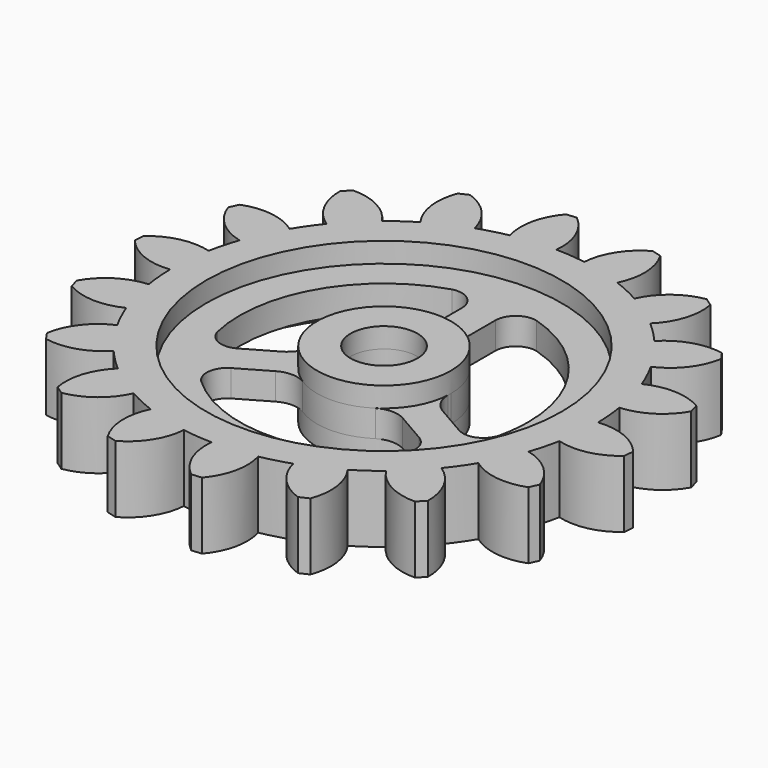
from build123d import *
from build123d import SkipClean  # not in build123d's __all__

# Parameters (mm, degrees)
F2_R      = 2.5
F4_DEPTH  = 5
F5_COUNT  = 18
F5_ANGLE  = 340
F7_DEPTH  = 5.001
F6_R      = 13.27
F6_W      = 2.5
F6_H      = 2.618576711
F8_DEPTH  = 1.5
F9_DEPTH  = 5.001
F10_START = 3.5
F10_DEPTH = 1.5
F11_R     = 5
F11_R_2   = 2.5
F12_DEPTH = 5


# Not quite as in the source:
# - a feature names something its author has since deleted; it is built from what else it names


with BuildPart() as f4:
    # F2 (on Top) → F4 (new body)
    with BuildSketch(Plane.XY):
        with BuildLine():
            ThreePointArc((-2.990858108, 15.4837872556), (-1.3744460631, 15.7099903889), (0.2566888126, 15.7679107955))
            ThreePointArc((0.2566888126, 15.7679107955), (-0.0491419998, 17.9196352526), (-1.341787956, 19.666780655))
            Line((-1.341787956, 19.666780655), (-2.0936974393, 19.6009970992))
            ThreePointArc((-2.0936974393, 19.6009970992), (-3.0633165837, 17.6559291466), (-2.990858108, 15.4837872556))
        make_face()
        with BuildLine():
            ThreePointArc((-2.990858108, 15.4837872556), (-10.0381040948, -12.1626216821), (15.77, 0))
            ThreePointArc((15.77, 0), (11.2414608164, 11.0599484046), (0.2566888126, 15.7679107955))
            ThreePointArc((0.2566888126, 15.7679107955), (-1.3744460631, 15.7099903889), (-2.990858108, 15.4837872556))
        make_face()
        Circle(F2_R, mode=Mode.SUBTRACT)
    extrude(amount=F4_DEPTH)

    # F5: F4 ×18 about axis
    f5_axis = Axis((0, 0, 30.7848658413), (0, 0, 1))


with BuildPart() as f4_1:
    add(f4.part, clean=False)
    for i in range(1, F5_COUNT):
        add(f4.part.rotate(f5_axis, i * F5_ANGLE / (F5_COUNT - 1)), clean=False)

    # F6 (on Top) → F7 (cut, through all)
    with BuildSketch(Plane.XY):
        with BuildLine():
            ThreePointArc((2.2618683613, 4.4591424642), (4.2608298374, 2.6163579833), (5, 0))
            ThreePointArc((5, 0), (4.9981658722, -0.1354175543), (4.9926648344, -0.2707357593))
            ThreePointArc((4.9926648344, -0.2707357593), (5.2571580162, -1.2784847908), (5.9926180702, -2.0164639659))
            Line((5.9926180702, -2.0164639659), (8.2603720268, -3.325752316))
            ThreePointArc((8.2603720268, -3.325752316), (9.5998090611, -3.4180506459), (10.4951545309, -2.4175672426))
            ThreePointArc((10.4951545309, -2.4175672426), (10.7010680378, -1.2165701176), (10.77, 0))
            ThreePointArc((10.77, 0), (8.6591117019, 6.4041146566), (3.1539025934, 10.2978540692))
            ThreePointArc((3.1539025934, 10.2978540692), (1.8397858158, 10.0227038458), (1.25, 8.8165681809))
            Line((1.25, 8.8165681809), (1.25, 6.1979914699))
            ThreePointArc((1.25, 6.1979914699), (1.5213786885, 5.1920747928), (2.2618683613, 4.4591424642))
        make_face()
        with BuildLine():
            ThreePointArc((-4.9926648325, -0.2707357951), (-4.3301270249, 2.4999999896), (-2.2618683613, 4.4591424642))
            ThreePointArc((-2.2618683613, 4.4591424642), (-1.5213786885, 5.1920747928), (-1.25, 6.1979914699))
            Line((-1.25, 6.1979914699), (-1.25, 8.8165681809))
            ThreePointArc((-1.25, 8.8165681809), (-1.8397858158, 10.0227038458), (-3.1539025934, 10.2978540692))
            ThreePointArc((-3.1539025934, 10.2978540692), (-9.3270936116, 5.3849999777), (-10.4951545136, -2.4175673179))
            ThreePointArc((-10.4951545136, -2.4175673179), (-9.5998090366, -3.4180507148), (-8.260372003, -3.3257523753))
            Line((-8.260372003, -3.3257523753), (-5.9926180557, -2.0164640089))
            ThreePointArc((-5.9926180557, -2.0164640089), (-5.257158007, -1.2784848286), (-4.9926648325, -0.2707357951))
        make_face()
    extrude(amount=F7_DEPTH, mode=Mode.SUBTRACT)

    # F6 (on Top) → F8 (cut)
    with BuildSketch(Plane.XY):
        Circle(F6_R)
        with BuildLine():
            ThreePointArc((-3.1539025934, 10.2978540692), (0, 10.77), (3.1539025934, 10.2978540692))
            ThreePointArc((3.1539025934, 10.2978540692), (8.6591117019, 6.4041146566), (10.77, 0))
            ThreePointArc((10.77, 0), (10.7010680378, -1.2165701176), (10.4951545309, -2.4175672426))
            ThreePointArc((10.4951545309, -2.4175672426), (9.3270936116, -5.3849999777), (7.3412519506, -7.880286784))
            ThreePointArc((7.3412519506, -7.880286784), (3.87e-08, -10.77), (-7.341251894, -7.8802868367))
            ThreePointArc((-7.341251894, -7.8802868367), (-9.327093573, -5.3850000446), (-10.4951545136, -2.4175673179))
            ThreePointArc((-10.4951545136, -2.4175673179), (-9.3270936116, 5.3849999777), (-3.1539025934, 10.2978540692))
        make_face(mode=Mode.SUBTRACT)
        with BuildLine():
            ThreePointArc((4.9926648344, -0.2707357593), (4.9981658722, -0.1354175543), (5, 0))
            ThreePointArc((5, 0), (4.2608298374, 2.6163579833), (2.2618683613, 4.4591424642))
            ThreePointArc((2.2618683613, 4.4591424642), (0, 5), (-2.2618683613, 4.4591424642))
            ThreePointArc((-2.2618683613, 4.4591424642), (-4.3301270249, 2.4999999896), (-4.9926648325, -0.2707357951))
            ThreePointArc((-4.9926648325, -0.2707357951), (-4.330127007, -2.5000000207), (-2.7307964524, -4.1884067061))
            ThreePointArc((-2.7307964524, -4.1884067061), (1.79e-08, -5), (2.7307964825, -4.1884066865))
            ThreePointArc((2.7307964825, -4.1884066865), (4.3301270249, -2.4999999896), (4.9926648344, -0.2707357593))
        make_face()
        with BuildLine():
            ThreePointArc((-2.2618683613, 4.4591424642), (0, 5), (2.2618683613, 4.4591424642))
            ThreePointArc((2.2618683613, 4.4591424642), (1.5213786885, 5.1920747928), (1.25, 6.1979914699))
            Line((1.25, 6.1979914699), (-1.25, 6.1979914699))
            ThreePointArc((-1.25, 6.1979914699), (-1.5213786885, 5.1920747928), (-2.2618683613, 4.4591424642))
        make_face()
        with Locations((0, 7.5072798254)):
            Rectangle(F6_W, F6_H)
        with BuildLine():
            Line((-1.25, 8.8165681809), (1.25, 8.8165681809))
            ThreePointArc((1.25, 8.8165681809), (1.8397858158, 10.0227038458), (3.1539025934, 10.2978540692))
            ThreePointArc((3.1539025934, 10.2978540692), (0, 10.77), (-3.1539025934, 10.2978540692))
            ThreePointArc((-3.1539025934, 10.2978540692), (-1.8397858158, 10.0227038458), (-1.25, 8.8165681809))
        make_face()
        with BuildLine():
            ThreePointArc((-2.7307964524, -4.1884067061), (-4.330127007, -2.5000000207), (-4.9926648325, -0.2707357951))
            ThreePointArc((-4.9926648325, -0.2707357951), (-5.257158007, -1.2784848286), (-5.9926180557, -2.0164640089))
            Line((-5.9926180557, -2.0164640089), (-4.7426180454, -4.1815275124))
            ThreePointArc((-4.7426180454, -4.1815275124), (-3.7357793059, -3.9135900073), (-2.7307964524, -4.1884067061))
        make_face()
        Polygon((-4.7426180454, -4.1815275124), (-5.9926180557, -2.0164640089), (-8.260372003, -3.3257523753), (-7.0103719926, -5.4908158787), align=None)
        with BuildLine():
            Line((-7.0103719926, -5.4908158787), (-8.260372003, -3.3257523753))
            ThreePointArc((-8.260372003, -3.3257523753), (-9.5998090366, -3.4180507148), (-10.4951545136, -2.4175673179))
            ThreePointArc((-10.4951545136, -2.4175673179), (-9.327093573, -5.3850000446), (-7.341251894, -7.8802868367))
            ThreePointArc((-7.341251894, -7.8802868367), (-7.7600232055, -6.6046532141), (-7.0103719926, -5.4908158787))
        make_face()
        with BuildLine():
            ThreePointArc((10.4951545309, -2.4175672426), (9.5998090611, -3.4180506459), (8.2603720268, -3.325752316))
            Line((8.2603720268, -3.325752316), (7.010372032, -5.4908158284))
            ThreePointArc((7.010372032, -5.4908158284), (7.7600232529, -6.6046531583), (7.3412519506, -7.880286784))
            ThreePointArc((7.3412519506, -7.880286784), (9.3270936116, -5.3849999777), (10.4951545309, -2.4175672426))
        make_face()
        Polygon((8.2603720268, -3.325752316), (5.9926180702, -2.0164639659), (4.7426180754, -4.1815274783), (7.010372032, -5.4908158284), align=None)
        with BuildLine():
            ThreePointArc((5.9926180702, -2.0164639659), (5.2571580162, -1.2784847908), (4.9926648344, -0.2707357593))
            ThreePointArc((4.9926648344, -0.2707357593), (4.3301270249, -2.4999999896), (2.7307964825, -4.1884066865))
            ThreePointArc((2.7307964825, -4.1884066865), (3.735779334, -3.9135899804), (4.7426180754, -4.1815274783))
            Line((4.7426180754, -4.1815274783), (5.9926180702, -2.0164639659))
        make_face()
    extrude(amount=F8_DEPTH, mode=Mode.SUBTRACT)

    # F9 (cut, through all): a face of the model
    f9_faces = [f4_1.faces().sort_by_distance(p)[0] for p in [
        (2.61e-08, -7.2727720269, 0),
    ]]
    extrude(f9_faces, amount=-F9_DEPTH, mode=Mode.SUBTRACT)

    # F6 (on Top) → F10 (cut)
    with BuildSketch(Plane.XY.offset(F10_START)):
        Circle(F6_R)
        with BuildLine():
            ThreePointArc((-3.1539025934, 10.2978540692), (0, 10.77), (3.1539025934, 10.2978540692))
            ThreePointArc((3.1539025934, 10.2978540692), (8.6591117019, 6.4041146566), (10.77, 0))
            ThreePointArc((10.77, 0), (10.7010680378, -1.2165701176), (10.4951545309, -2.4175672426))
            ThreePointArc((10.4951545309, -2.4175672426), (9.3270936116, -5.3849999777), (7.3412519506, -7.880286784))
            ThreePointArc((7.3412519506, -7.880286784), (3.87e-08, -10.77), (-7.341251894, -7.8802868367))
            ThreePointArc((-7.341251894, -7.8802868367), (-9.327093573, -5.3850000446), (-10.4951545136, -2.4175673179))
            ThreePointArc((-10.4951545136, -2.4175673179), (-9.3270936116, 5.3849999777), (-3.1539025934, 10.2978540692))
        make_face(mode=Mode.SUBTRACT)
        with BuildLine():
            ThreePointArc((4.9926648344, -0.2707357593), (4.9981658722, -0.1354175543), (5, 0))
            ThreePointArc((5, 0), (4.2608298374, 2.6163579833), (2.2618683613, 4.4591424642))
            ThreePointArc((2.2618683613, 4.4591424642), (0, 5), (-2.2618683613, 4.4591424642))
            ThreePointArc((-2.2618683613, 4.4591424642), (-4.3301270249, 2.4999999896), (-4.9926648325, -0.2707357951))
            ThreePointArc((-4.9926648325, -0.2707357951), (-4.330127007, -2.5000000207), (-2.7307964524, -4.1884067061))
            ThreePointArc((-2.7307964524, -4.1884067061), (1.79e-08, -5), (2.7307964825, -4.1884066865))
            ThreePointArc((2.7307964825, -4.1884066865), (4.3301270249, -2.4999999896), (4.9926648344, -0.2707357593))
        make_face()
        with BuildLine():
            ThreePointArc((10.4951545309, -2.4175672426), (9.5998090611, -3.4180506459), (8.2603720268, -3.325752316))
            Line((8.2603720268, -3.325752316), (7.010372032, -5.4908158284))
            ThreePointArc((7.010372032, -5.4908158284), (7.7600232529, -6.6046531583), (7.3412519506, -7.880286784))
            ThreePointArc((7.3412519506, -7.880286784), (9.3270936116, -5.3849999777), (10.4951545309, -2.4175672426))
        make_face()
        Polygon((8.2603720268, -3.325752316), (5.9926180702, -2.0164639659), (4.7426180754, -4.1815274783), (7.010372032, -5.4908158284), align=None)
        with BuildLine():
            ThreePointArc((5.9926180702, -2.0164639659), (5.2571580162, -1.2784847908), (4.9926648344, -0.2707357593))
            ThreePointArc((4.9926648344, -0.2707357593), (4.3301270249, -2.4999999896), (2.7307964825, -4.1884066865))
            ThreePointArc((2.7307964825, -4.1884066865), (3.735779334, -3.9135899804), (4.7426180754, -4.1815274783))
            Line((4.7426180754, -4.1815274783), (5.9926180702, -2.0164639659))
        make_face()
        with BuildLine():
            ThreePointArc((-2.2618683613, 4.4591424642), (0, 5), (2.2618683613, 4.4591424642))
            ThreePointArc((2.2618683613, 4.4591424642), (1.5213786885, 5.1920747928), (1.25, 6.1979914699))
            Line((1.25, 6.1979914699), (-1.25, 6.1979914699))
            ThreePointArc((-1.25, 6.1979914699), (-1.5213786885, 5.1920747928), (-2.2618683613, 4.4591424642))
        make_face()
        with Locations((0, 7.5072798254)):
            Rectangle(F6_W, F6_H)
        with BuildLine():
            Line((-1.25, 8.8165681809), (1.25, 8.8165681809))
            ThreePointArc((1.25, 8.8165681809), (1.8397858158, 10.0227038458), (3.1539025934, 10.2978540692))
            ThreePointArc((3.1539025934, 10.2978540692), (0, 10.77), (-3.1539025934, 10.2978540692))
            ThreePointArc((-3.1539025934, 10.2978540692), (-1.8397858158, 10.0227038458), (-1.25, 8.8165681809))
        make_face()
        with BuildLine():
            ThreePointArc((-2.7307964524, -4.1884067061), (-4.330127007, -2.5000000207), (-4.9926648325, -0.2707357951))
            ThreePointArc((-4.9926648325, -0.2707357951), (-5.257158007, -1.2784848286), (-5.9926180557, -2.0164640089))
            Line((-5.9926180557, -2.0164640089), (-4.7426180454, -4.1815275124))
            ThreePointArc((-4.7426180454, -4.1815275124), (-3.7357793059, -3.9135900073), (-2.7307964524, -4.1884067061))
        make_face()
        Polygon((-4.7426180454, -4.1815275124), (-5.9926180557, -2.0164640089), (-8.260372003, -3.3257523753), (-7.0103719926, -5.4908158787), align=None)
        with BuildLine():
            Line((-7.0103719926, -5.4908158787), (-8.260372003, -3.3257523753))
            ThreePointArc((-8.260372003, -3.3257523753), (-9.5998090366, -3.4180507148), (-10.4951545136, -2.4175673179))
            ThreePointArc((-10.4951545136, -2.4175673179), (-9.327093573, -5.3850000446), (-7.341251894, -7.8802868367))
            ThreePointArc((-7.341251894, -7.8802868367), (-7.7600232055, -6.6046532141), (-7.0103719926, -5.4908158787))
        make_face()
    extrude(amount=F10_DEPTH, mode=Mode.SUBTRACT)

    # F11 (on Top) → F12 (join)
    with BuildSketch(Plane.XY):
        Circle(F11_R)
        Circle(F11_R_2, mode=Mode.SUBTRACT)
    with SkipClean():  # cleaning this boolean's faces spoils the solid; the shape is the same uncleaned
        extrude(amount=F12_DEPTH)


solid = f4_1.part
